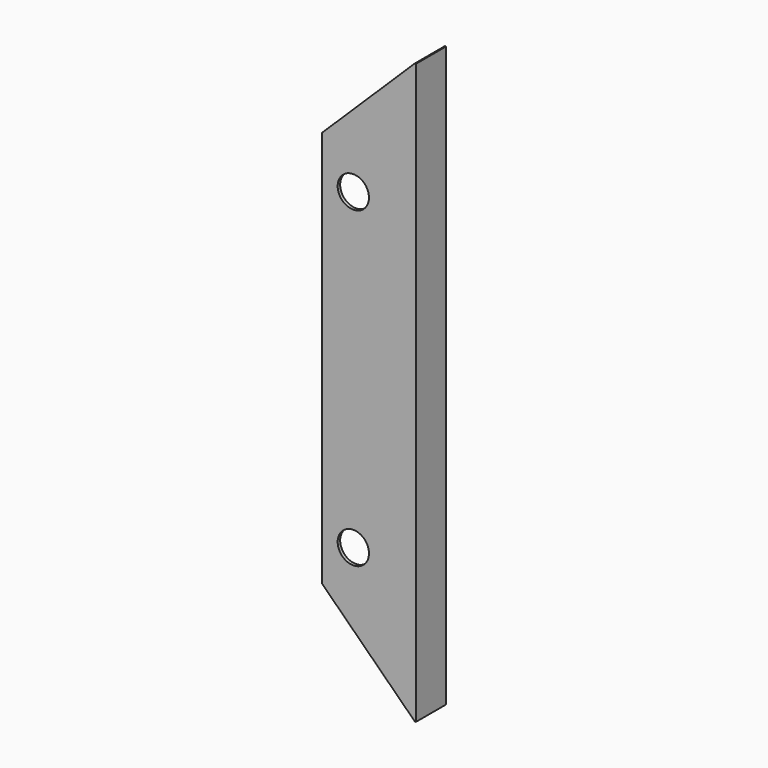
from build123d import *

# Parameters (mm, degrees)
F1_DEPTH = 1850
F3_DEPTH = 200
F4_R     = 50
F5_DEPTH = 120.001


# Not quite as in the source:
# - a feature names something its author has since deleted; it is built from what else it names


with BuildPart() as f1:
    # F0 (on Top) → F1 (new body)
    with BuildSketch(Plane.XY):
        Polygon((-100, 0), (-110, 0), (-110, -30), (190, -30), (190, 90), (180, 90), (180, -20), (-100, -20), align=None)
    extrude(amount=F1_DEPTH)

    # F2 (on face) → F3 (cut)
    with BuildSketch(Plane.XZ.offset(30)):
        Polygon((186.4785214056, 0), (-110, 291.3486315578), (-110, 0), align=None)
        Polygon((-110, 1850), (-110, 1558.6513684422), (186.4785214056, 1850), align=None)
    extrude(amount=-F3_DEPTH, mode=Mode.SUBTRACT)

    # F4 (on face) → F5 (cut, through all)
    with BuildSketch(Plane.XZ.offset(30)):
        with Locations((-10, 425)):
            Circle(F4_R)
        with Locations((-10, 1425)):
            Circle(F4_R)
    extrude(amount=-F5_DEPTH, mode=Mode.SUBTRACT)


solid = f1.part
